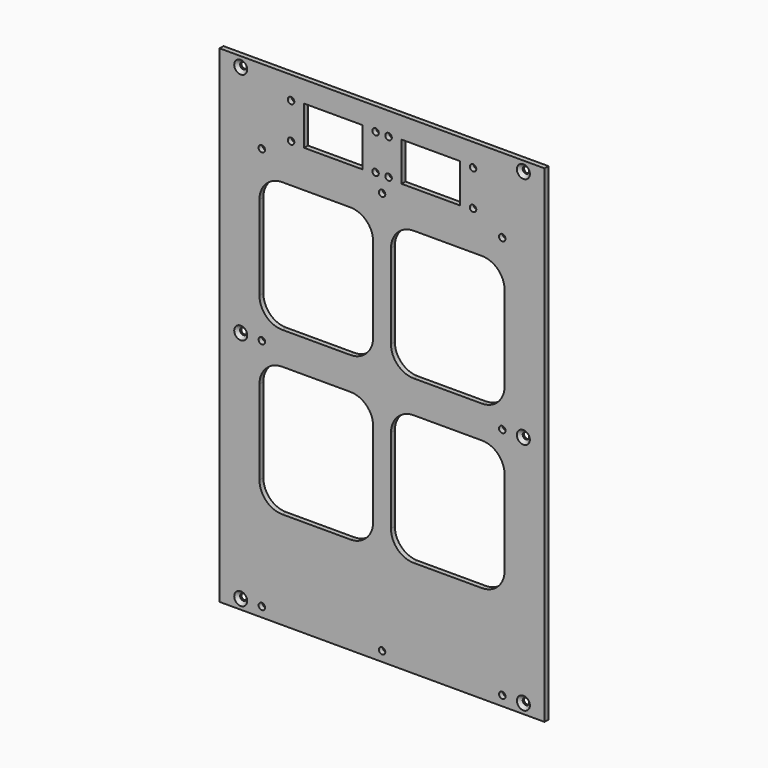
from build123d import *

# Parameters (mm, degrees)
F0_W           = 100
F0_H           = 150
F1_DEPTH       = 1.5
F3_D           = 2
F3_CSINK_D     = 4
F3_CSINK_ANGLE = 90
F4_D           = 2
F6_D           = 2


# Not quite as in the source:
# - a feature names something its author has since deleted; it is built from what else it names


with BuildPart() as f1:
    # F0 (on Front) → F1 (new body)
    with BuildSketch(Plane.XZ):
        Rectangle(F0_W, F0_H)
        with BuildLine():
            Line((-30.7377611669, -5), (-9.7377611669, -5))
            ThreePointArc((-9.7377611669, -5), (-4.7880136986, -7.0502525317), (-2.7377611669, -12))
            Line((-2.7377611669, -12), (-2.7377611669, -38))
            ThreePointArc((-2.7377611669, -38), (-4.7880136986, -42.9497474683), (-9.7377611669, -45))
            Line((-9.7377611669, -45), (-30.7377611669, -45))
            ThreePointArc((-30.7377611669, -45), (-35.6875086352, -42.9497474683), (-37.7377611669, -38))
            Line((-37.7377611669, -38), (-37.7377611669, -12))
            ThreePointArc((-37.7377611669, -12), (-35.6875086352, -7.0502525317), (-30.7377611669, -5))
        make_face(mode=Mode.SUBTRACT)
        with BuildLine():
            ThreePointArc((37.7377611669, -38), (35.6875086352, -42.9497474683), (30.7377611669, -45))
            Line((30.7377611669, -45), (9.7377611669, -45))
            ThreePointArc((9.7377611669, -45), (4.7880136986, -42.9497474683), (2.7377611669, -38))
            Line((2.7377611669, -38), (2.7377611669, -12))
            ThreePointArc((2.7377611669, -12), (4.7880136986, -7.0502525317), (9.7377611669, -5))
            Line((9.7377611669, -5), (30.7377611669, -5))
            ThreePointArc((30.7377611669, -5), (35.6875086352, -7.0502525317), (37.7377611669, -12))
            Line((37.7377611669, -12), (37.7377611669, -38))
        make_face(mode=Mode.SUBTRACT)
        with BuildLine():
            ThreePointArc((-2.7377611669, 12), (-4.7880136986, 7.0502525317), (-9.7377611669, 5))
            Line((-9.7377611669, 5), (-30.7377611669, 5))
            ThreePointArc((-30.7377611669, 5), (-35.6875086352, 7.0502525317), (-37.7377611669, 12))
            Line((-37.7377611669, 12), (-37.7377611669, 38))
            ThreePointArc((-37.7377611669, 38), (-35.6875086352, 42.9497474683), (-30.7377611669, 45))
            Line((-30.7377611669, 45), (-9.7377611669, 45))
            ThreePointArc((-9.7377611669, 45), (-4.7880136986, 42.9497474683), (-2.7377611669, 38))
            Line((-2.7377611669, 38), (-2.7377611669, 12))
        make_face(mode=Mode.SUBTRACT)
        Polygon((-24, 56.5), (-24, 68.5), (-15, 68.5), (-6, 68.5), (-6, 56.5), (-15, 56.5), align=None, mode=Mode.SUBTRACT)
        with BuildLine():
            ThreePointArc((9.7377611669, 5), (4.7880136986, 7.0502525317), (2.7377611669, 12))
            Line((2.7377611669, 12), (2.7377611669, 38))
            ThreePointArc((2.7377611669, 38), (4.7880136986, 42.9497474683), (9.7377611669, 45))
            Line((9.7377611669, 45), (30.7377611669, 45))
            ThreePointArc((30.7377611669, 45), (35.6875086352, 42.9497474683), (37.7377611669, 38))
            Line((37.7377611669, 38), (37.7377611669, 12))
            ThreePointArc((37.7377611669, 12), (35.6875086352, 7.0502525317), (30.7377611669, 5))
            Line((30.7377611669, 5), (9.7377611669, 5))
        make_face(mode=Mode.SUBTRACT)
        Polygon((6, 56.5), (6, 68.5), (15, 68.5), (24, 68.5), (24, 56.5), (15, 56.5), align=None, mode=Mode.SUBTRACT)
    extrude(amount=F1_DEPTH)

    # F3 (through all)
    with Locations(Plane.XZ.offset(1.5)):
        with Locations((-43.5, -72), (43.5, -72), (43.5, 72), (-43.5, 72), (-43.5, 0), (43.5, 0)):
            CounterSinkHole(F3_D / 2, F3_CSINK_D / 2, counter_sink_angle=F3_CSINK_ANGLE)

    # F4 (through all)
    with Locations(Plane(origin=(0, 0, 0), x_dir=(1, 0, 0), z_dir=(0, 1, 0))):
        with Locations((-28, -68), (-28, -57), (-2, -57), (-2, -68), (2, -68), (2, -57), (28, -57), (28, -68)):
            Hole(F4_D / 2)

    # F6 (through all)
    with Locations(Plane(origin=(0, 0, 0), x_dir=(1, 0, 0), z_dir=(0, 1, 0))):
        with Locations((-37, 72), (0, 72), (37, 72), (0, -52), (-37, -52), (37, -52), (-37, 0), (37, 0)):
            Hole(F6_D / 2)


solid = f1.part
